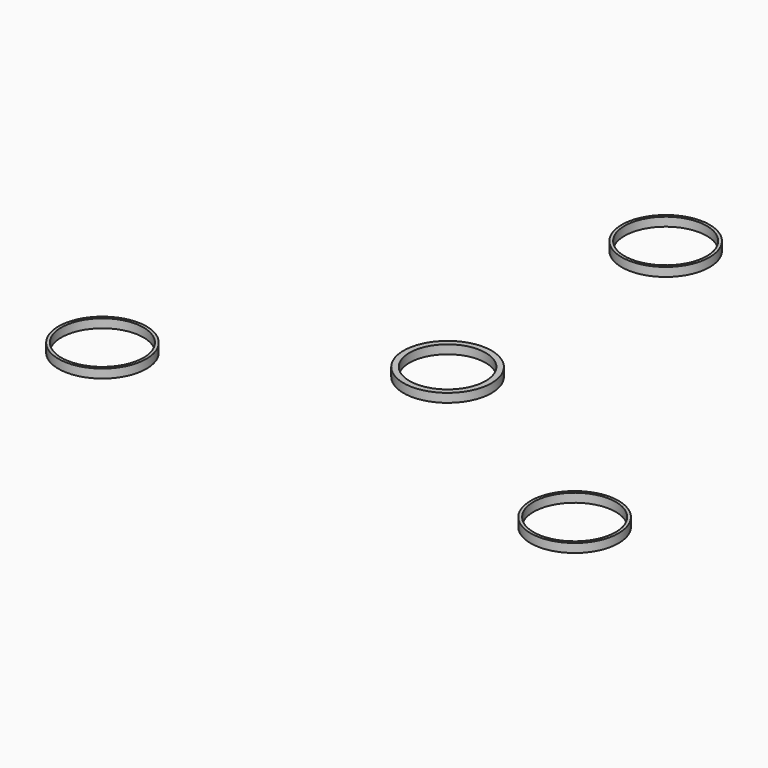
from build123d import *

# Parameters (mm, degrees)
F0_R     = 15
F0_R_2   = 14
F1_DEPTH = 3
F0_R_3   = 13


# Not quite as in the source:
# - a feature names something its author has since deleted; it is built from what else it names


with BuildPart() as f1:
    # F0 (on Top) → F1 (new body)
    with BuildSketch(Plane.XY):
        with Locations((0, 92.926489729)):
            Circle(F0_R)
        with Locations((0, 92.926489729)):
            Circle(F0_R_2, mode=Mode.SUBTRACT)
    extrude(amount=F1_DEPTH)


with BuildPart() as f1b:
    # F0 (on Top) → F1, piece 2 (new body)
    with BuildSketch(Plane.XY):
        with Locations((80.4767007898, -46.4632448645)):
            Circle(F0_R)
        with Locations((80.4767007898, -46.4632448645)):
            Circle(F0_R_2, mode=Mode.SUBTRACT)
    extrude(amount=F1_DEPTH)


with BuildPart() as f1c:
    # F0 (on Top) → F1, piece 3 (new body)
    with BuildSketch(Plane.XY):
        Circle(F0_R)
        Circle(F0_R_3, mode=Mode.SUBTRACT)
    extrude(amount=F1_DEPTH)


with BuildPart() as f1d:
    # F0 (on Top) → F1, piece 4 (new body)
    with BuildSketch(Plane.XY):
        with Locations((-80.4767007898, -46.4632448645)):
            Circle(F0_R)
        with Locations((-80.4767007898, -46.4632448645)):
            Circle(F0_R_2, mode=Mode.SUBTRACT)
    extrude(amount=F1_DEPTH)


solid = Compound([f1.part, f1b.part, f1c.part, f1d.part])
